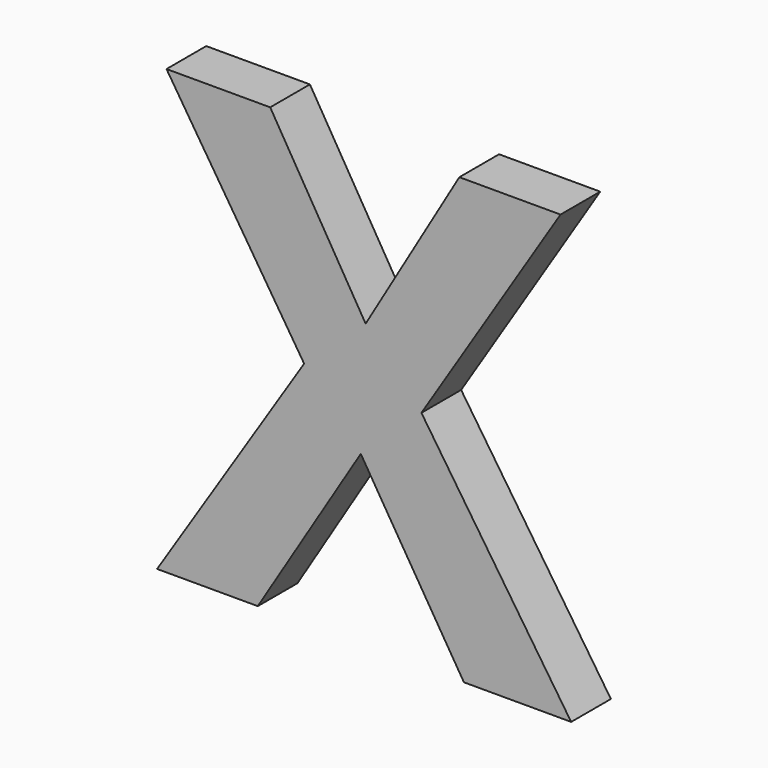
from build123d import *

# Parameters (mm, degrees)
F0_TEXT_SIZE = 62.5
F1_DEPTH     = 5


# Not quite as in the source:
# - Text() gives the source's letters only with a copy of the font that has no kerning and outlines rounded to 1/6400 em; it was checked with that copy


with BuildPart() as f1:
    # F0 (on Front) → F1 (new body)
    with BuildSketch(Plane.XZ):
        with Locations((-62.782255169, 20.0806437765)):
            Text('X', F0_TEXT_SIZE, font='Open Sans', font_style=FontStyle.BOLD, text_align=(TextAlign.LEFT, TextAlign.BOTTOM))
    extrude(amount=F1_DEPTH)


solid = f1.part
